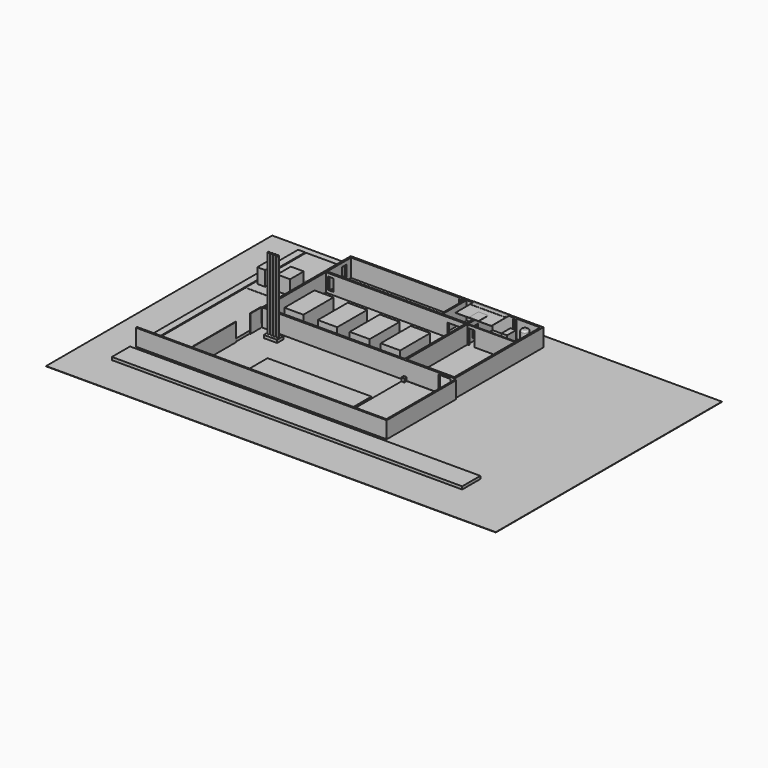
from build123d import *

# Parameters (mm, degrees)
F0_W        = 75397.331237793
F0_H        = 47390.0489807129
F1_DEPTH    = 25
F2_W        = 23400
F2_H        = 12700
F2_H_2      = 5000
F3_DEPTH    = 3000
F4_W        = 8300
F4_H        = 14000
F5_DEPTH    = 200
F2_W_2      = 1173.3947754007
F2_H_3      = 33162.7039081701
F2_W_3      = 58729.1374206543
F2_H_4      = 3803.1048774719
F2_W_4      = 8000
F2_H_5      = 33131.3623554357
F2_W_5      = 2231.9564819336
F2_H_6      = 1301.4698028564
F3_FACE_W   = 75397.331237793
F3_FACE_H   = 47390.0489807129
F3_FACE_W_2 = 32300
F3_FACE_H_2 = 18600
F6_DEPTH    = 25
F7_DEPTH    = 200
F8_W        = 17412.4488830566
F8_H        = 7584.0892791748
F9_DEPTH    = 200
F10_W       = 2000
F10_H       = 2500
F11_DEPTH   = 400
F12_W       = 1200
F12_H       = 2200
F13_DEPTH   = 310
F14_W       = 977.3139953613
F14_H       = 2184.4711005688
F15_DEPTH   = 305
F16_W       = 500
F16_H       = 500
F16_W_2     = 455.0476074219
F17_DEPTH   = 600
F18_W       = 912.5473359871
F18_H       = 2500
F19_DEPTH   = 310
F20_W       = 300
F20_H       = 300
F20_H_2     = 21.6979980468
F21_DEPTH   = 3000
F22_W       = 2000
F22_H       = 2200
F23_DEPTH   = 8200.202237882
F24_W       = 7344.9523925781
F24_H       = 250
F25_DEPTH   = 1000
F27_W       = 110.0954055786
F27_H       = 2346.9123840332
F28_DEPTH   = 3000
F29_W       = 8000
F29_H       = 150
F30_DEPTH   = 3000
F31_W       = 1000
F31_H       = 2500
F32_DEPTH   = 250
F33_DEPTH   = 500
F34_R       = 175
F35_DEPTH   = 12000
F36_W       = 8000
F36_H       = 6500.6484985352
F37_DEPTH   = 25
F38_W       = 2166.8834686279
F38_H       = 2863.3804321289
F38_W_2     = 1315.6070709229
F38_H_2     = 2940.7691955566
F39_DEPTH   = 2500
F40_DEPTH   = 2800
F41_W       = 923.1796264648
F41_H       = 1872.3831176758
F41_W_2     = 2271.7437744141
F41_H_2     = 921.8673706055
F42_DEPTH   = 1500
F43_R       = 618.5809959927
F44_DEPTH   = 2500
F45_R       = 300
F46_W       = 230.0758361816
F46_H       = 5000
F47_DEPTH   = 3000
F49_W       = 6000
F49_H       = 4000
F50_DEPTH   = 25
F51_W       = 5631.3896179199
F51_H       = 600.0671386719
F51_W_2     = 819.3206787109
F51_H_2     = 2024.5748645909
F52_DEPTH   = 25
F53_W       = 3182.8193664551
F53_H       = 6288.0077362061
F53_W_2     = 3260.4484558105
F53_W_3     = 3338.0794525146
F54_DEPTH   = 3000


with BuildPart() as f1:
    # F0 (on Top) → F1 (new body)
    with BuildSketch(Plane.XY):
        with Locations((37698.6656188965, 23695.0244903564)):
            Rectangle(F0_W, F0_H)
    extrude(amount=F1_DEPTH)

    # F2 (on face) → F3 (join)
    with BuildSketch(Plane.XY.offset(25)):
        Polygon((15250.3890991211, 44789.8477428309), (15250.3890991211, 44489.8477428309), (15250.3890991211, 39489.8477428309), (15250.3890991211, 39189.8477428309), (15250.3890991211, 26489.8477428309), (15250.3890991211, 26189.8477428309), (47550.3890991211, 26189.8477428309), (47550.3890991211, 44789.8477428309), align=None)
        with Locations((27250.3890991211, 32839.8477428309)):
            Rectangle(F2_W, F2_H, mode=Mode.SUBTRACT)
        with Locations((27250.3890991211, 41989.8477428309)):
            Rectangle(F2_W, F2_H_2, mode=Mode.SUBTRACT)
        Polygon((39250.3890991211, 44489.8477428309), (47250.3890991211, 44489.8477428309), (47250.3890991211, 26489.8477428309), (39250.3890991211, 26489.8477428309), (39250.3890991211, 39189.8477428309), align=None, mode=Mode.SUBTRACT)
    extrude(amount=F3_DEPTH)

    # F2 (on face) + F3_face (on face) → F6 (join)
    with BuildSketch(Plane.XY.offset(25)):
        Polygon((15250.3890991211, 44789.8477428309), (15250.3890991211, 44489.8477428309), (15250.3890991211, 39489.8477428309), (15250.3890991211, 39189.8477428309), (15250.3890991211, 26489.8477428309), (15250.3890991211, 26189.8477428309), (47550.3890991211, 26189.8477428309), (47550.3890991211, 44789.8477428309), align=None)
        with Locations((27250.3890991211, 32839.8477428309)):
            Rectangle(F2_W, F2_H, mode=Mode.SUBTRACT)
        with Locations((27250.3890991211, 41989.8477428309)):
            Rectangle(F2_W, F2_H_2, mode=Mode.SUBTRACT)
        Polygon((39250.3890991211, 44489.8477428309), (47250.3890991211, 44489.8477428309), (47250.3890991211, 26489.8477428309), (39250.3890991211, 26489.8477428309), (39250.3890991211, 39189.8477428309), align=None, mode=Mode.SUBTRACT)
        with Locations((6325.022983546, 29071.1996969159)):
            Rectangle(F2_W_2, F2_H_3)
        with Locations((35048.9876026129, 8588.2953040949)):
            Rectangle(F2_W_3, F2_H_4)
        with Locations((11100.3890991211, 29055.5289205487)):
            Rectangle(F2_W_4, F2_H_5)
        with Locations((18424.6368408203, 24639.702796936)):
            Rectangle(F2_W_5, F2_H_6)
    with BuildSketch(Plane(origin=(38971.7115657614, 21310.9830961107, 25), x_dir=(1, 0, 0), z_dir=(0, 0, 1))):
        with Locations((-1273.0459468649, 2384.0413942457)):
            Rectangle(F3_FACE_W, F3_FACE_H)
        with Locations((-7571.3224666403, 14178.8646467202)):
            Rectangle(F3_FACE_W_2, F3_FACE_H_2, mode=Mode.SUBTRACT)
    extrude(amount=F6_DEPTH)

    # F2 (on face) → F7 (join)
    with BuildSketch(Plane.XY.offset(25)):
        Polygon((15250.3890991211, 44789.8477428309), (15250.3890991211, 44489.8477428309), (15250.3890991211, 39489.8477428309), (15250.3890991211, 39189.8477428309), (15250.3890991211, 26489.8477428309), (15250.3890991211, 26189.8477428309), (47550.3890991211, 26189.8477428309), (47550.3890991211, 44789.8477428309), align=None)
        with Locations((27250.3890991211, 32839.8477428309)):
            Rectangle(F2_W, F2_H, mode=Mode.SUBTRACT)
        with Locations((27250.3890991211, 41989.8477428309)):
            Rectangle(F2_W, F2_H_2, mode=Mode.SUBTRACT)
        Polygon((39250.3890991211, 44489.8477428309), (47250.3890991211, 44489.8477428309), (47250.3890991211, 26489.8477428309), (39250.3890991211, 26489.8477428309), (39250.3890991211, 39189.8477428309), align=None, mode=Mode.SUBTRACT)
        with Locations((6325.022983546, 29071.1996969159)):
            Rectangle(F2_W_2, F2_H_3)
        with Locations((35048.9876026129, 8588.2953040949)):
            Rectangle(F2_W_3, F2_H_4)
        with Locations((11100.3890991211, 29055.5289205487)):
            Rectangle(F2_W_4, F2_H_5)
        with Locations((18424.6368408203, 24639.702796936)):
            Rectangle(F2_W_5, F2_H_6)
    extrude(amount=F7_DEPTH)

    # F8 (on face) → F9 (join)
    with BuildSketch(Plane.XY.offset(50)):
        with Locations((30193.1591033936, 15763.8807296753)):
            Rectangle(F8_W, F8_H)
    extrude(amount=F9_DEPTH)

    # F10 (on face) → F11 (cut)
    with BuildSketch(Plane.XZ.offset(-26189.8477428309)):
        with Locations((45814.1078948975, 1479.7965964478)):
            Rectangle(F10_W, F10_H)
    extrude(amount=-F11_DEPTH, mode=Mode.SUBTRACT)

    # F12 (on face) → F13 (cut)
    with BuildSketch(Plane.YZ.offset(39250.3890991211)):
        with Locations((40870.0355529785, 1125)):
            Rectangle(F12_W, F12_H)
    extrude(amount=-F13_DEPTH, mode=Mode.SUBTRACT)

    # F14 (on face) → F15 (cut)
    with BuildSketch(Plane(origin=(15250.3890991211, 0, 0), x_dir=(0, -1, 0), z_dir=(-1, 0, 0))):
        with Locations((-43031.3739776611, 1313.1873756647)):
            Rectangle(F14_W, F14_H)
    extrude(amount=-F15_DEPTH, mode=Mode.SUBTRACT)

    # F18 (on face) → F19 (cut)
    with BuildSketch(Plane.XZ.offset(-39189.8477428309)):
        with Locations((16364.5578553104, 1275)):
            Rectangle(F18_W, F18_H)
    extrude(amount=-F19_DEPTH, mode=Mode.SUBTRACT)

    # F20 (on face) → F21 (join)
    with BuildSketch(Plane.XY.offset(25)):
        with Locations((43100.3890991211, 44339.8477428309)):
            Rectangle(F20_W, F20_H)
        with Locations((43100.3890991211, 39361.5457408778)):
            Rectangle(F20_W, F20_H)
        with Locations((33995.8290100098, 39500.6967418544)):
            Rectangle(F20_W, F20_H_2)
        with Locations((33995.8290100098, 44339.8477428309)):
            Rectangle(F20_W, F20_H)
    extrude(amount=F21_DEPTH)

    # F22 (on face) → F23 (cut, through all)
    with BuildSketch(Plane.XZ.offset(-39189.8477428309)):
        with Locations((36990.2000427246, 1125)):
            Rectangle(F22_W, F22_H)
    extrude(amount=-F23_DEPTH, mode=Mode.SUBTRACT)

    # F27 (on face) → F28 (join)
    with BuildSketch(Plane.XY.offset(50)):
        with Locations((15155.4368019104, 24997.2095489502)):
            Rectangle(F27_W, F27_H)
        Polygon((15210.4845046997, 20823.7533569336), (15100.3890991211, 20823.7533569336), (15100.3890991211, 12489.8477428309), (15100.3890991211, 11783.4882736206), (15210.4845046997, 11783.4882736206), align=None)
    extrude(amount=F28_DEPTH)

    # F29 (on face) → F30 (join)
    with BuildSketch(Plane.XY.offset(25)):
        with Locations((43250.3890991211, 39286.5457408778)):
            Rectangle(F29_W, F29_H)
    extrude(amount=F30_DEPTH)

    # F31 (on face) → F32 (cut)
    with BuildSketch(Plane.XZ.offset(-39211.5457408778)):
        with Locations((39965.4886870131, 1275)):
            Rectangle(F31_W, F31_H)
    extrude(amount=-F32_DEPTH, mode=Mode.SUBTRACT)

    # F2 (on face) → F33 (join)
    with BuildSketch(Plane.XY.offset(25)):
        Polygon((15250.3890991211, 44789.8477428309), (15250.3890991211, 44489.8477428309), (15250.3890991211, 39489.8477428309), (15250.3890991211, 39189.8477428309), (15250.3890991211, 26489.8477428309), (15250.3890991211, 26189.8477428309), (47550.3890991211, 26189.8477428309), (47550.3890991211, 44789.8477428309), align=None)
        with Locations((27250.3890991211, 32839.8477428309)):
            Rectangle(F2_W, F2_H, mode=Mode.SUBTRACT)
        with Locations((27250.3890991211, 41989.8477428309)):
            Rectangle(F2_W, F2_H_2, mode=Mode.SUBTRACT)
        Polygon((39250.3890991211, 44489.8477428309), (47250.3890991211, 44489.8477428309), (47250.3890991211, 26489.8477428309), (39250.3890991211, 26489.8477428309), (39250.3890991211, 39189.8477428309), align=None, mode=Mode.SUBTRACT)
        with Locations((6325.022983546, 29071.1996969159)):
            Rectangle(F2_W_2, F2_H_3)
        with Locations((35048.9876026129, 8588.2953040949)):
            Rectangle(F2_W_3, F2_H_4)
        with Locations((11100.3890991211, 29055.5289205487)):
            Rectangle(F2_W_4, F2_H_5)
        with Locations((18424.6368408203, 24639.702796936)):
            Rectangle(F2_W_5, F2_H_6)
    extrude(amount=F33_DEPTH)

    # F34 (on face) → F35 (join)
    with BuildSketch(Plane.XY.offset(525)):
        with Locations((17596.2409973145, 24665.5521392822)):
            Circle(F34_R)
        with Locations((18112.548828125, 24665.5521392822)):
            Circle(F34_R)
        with Locations((18598.1731414795, 24665.5521392822)):
            Circle(F34_R)
        with Locations((19108.4899902344, 24665.5521392822)):
            Circle(F34_R)
    extrude(amount=F35_DEPTH)

    # F36 (on face) → F37 (join)
    with BuildSketch(Plane.XY.offset(525)):
        with Locations((11100.3890991211, 36170.2842712402)):
            Rectangle(F36_W, F36_H)
    extrude(amount=F37_DEPTH)

    # F38 (on face) → F39 (join)
    with BuildSketch(Plane.XY.offset(525)):
        with Locations((12064.6305084229, 36131.5879821777)):
            Rectangle(F38_W, F38_H)
        with Locations((8311.2802505493, 36170.2823638916)):
            Rectangle(F38_W_2, F38_H_2)
    extrude(amount=F39_DEPTH)

    # F41 (on face) → F42 (join)
    with BuildSketch(Plane.XY.offset(25)):
        with Locations((42996.9139099121, 43219.7875976562)):
            Rectangle(F41_W, F41_H)
        with Locations((44959.3620300293, 40929.4548034668)):
            Rectangle(F41_W_2, F41_H_2)
    extrude(amount=F42_DEPTH)

    # F43 (on face) → F44 (join)
    with BuildSketch(Plane.XY.offset(25)):
        with Locations((45370.9106445312, 43629.1999816895)):
            Circle(F43_R)
    extrude(amount=F44_DEPTH)

    # F45
    f45_edges = [f1.edges().sort_by_distance(p)[0] for p in [
        (44752.329649, 43629.199982, 2525),
    ]]
    fillet(f45_edges, radius=F45_R)

    # F46 (on face) → F47 (join)
    with BuildSketch(Plane.XY.offset(25)):
        with Locations((34788.0802154541, 41989.8477428309)):
            Rectangle(F46_W, F46_H)
    extrude(amount=F47_DEPTH)

    # F49 (on face) → F50 (join)
    with BuildSketch(Plane.XY.offset(3025)):
        with Locations((39007.1907043457, 42789.8477428309)):
            Rectangle(F49_W, F49_H)
    extrude(amount=F50_DEPTH)

    # F51 (on face) → F52 (join)
    with BuildSketch(Plane.XY.offset(3050)):
        with Locations((39004.1675567627, 44129.9514770508)):
            Rectangle(F51_W, F51_H)
        with Locations((38652.2064208984, 41802.1351751264)):
            Rectangle(F51_W_2, F51_H_2)
        with Locations((39471.5270996094, 41802.1351751264)):
            Rectangle(F51_W_2, F51_H_2)
    extrude(amount=F52_DEPTH)

    # F53 (on face) → F54 (join)
    with BuildSketch(Plane.XY.offset(25)):
        with Locations((19197.5803375244, 31087.8801345825)):
            Rectangle(F53_W, F53_H)
        with Locations((24825.7369995117, 31087.8801345825)):
            Rectangle(F53_W_2, F53_H)
        with Locations((30221.0054397583, 31087.8801345825)):
            Rectangle(F53_W_3, F53_H)
        with Locations((35383.3827972412, 31087.8801345825)):
            Rectangle(F53_W_2, F53_H)
    extrude(amount=F54_DEPTH)


with BuildPart() as f5:
    # F4 (on face) → F5 (new body)
    with BuildSketch(Plane.XY.offset(25)):
        with Locations((43400.3890991211, 18889.8477428309)):
            Rectangle(F4_W, F4_H)
    extrude(amount=F5_DEPTH)

    # F16 (on face) → F17 (join)
    with BuildSketch(Plane.XY.offset(225)):
        with Locations((47300.3890991211, 12139.8477428309)):
            Rectangle(F16_W, F16_H)
        with Locations((39477.912902832, 12139.8477428309)):
            Rectangle(F16_W_2, F16_H)
        with Locations((39500.3890991211, 25639.8477428309)):
            Rectangle(F16_W, F16_H)
        with Locations((47300.3890991211, 25639.8477428309)):
            Rectangle(F16_W, F16_H)
    extrude(amount=F17_DEPTH)

    # F24 (on face) → F25 (join)
    with BuildSketch(Plane.XY.offset(225)):
        with Locations((43377.912902832, 12014.8477428309)):
            Rectangle(F24_W, F24_H)
    extrude(amount=F25_DEPTH)


with BuildPart() as f40:
    # F26 (on face) → F40 (new body)
    with BuildSketch(Plane.XY.offset(50)):
        Polygon((47550.3890991211, 11638.8477428309), (47800.3890991211, 11638.8477428309), (47800.3890991211, 11888.8477428309), (47800.3890991211, 26189.8477428309), (47550.3890991211, 26189.8477428309), (47550.3890991211, 11888.8477428309), (5738.3255958457, 11888.8477428309), (5738.3255958457, 11638.8477428309), align=None)
    extrude(amount=F40_DEPTH)


solid = Compound([f1.part, f5.part, f40.part])
